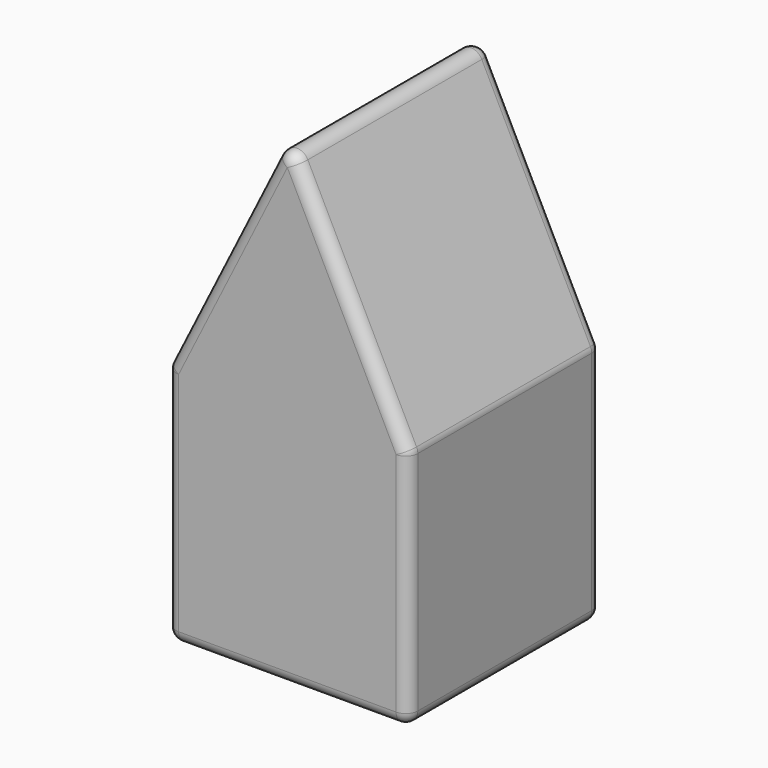
from build123d import *

# Parameters (mm, degrees)
F0_W     = 101.6
F0_H     = 101.6
F1_DEPTH = 101.6
F2_W     = 101.6
F2_H     = 101.6
F3_DEPTH = 101.6
F5_DEPTH = 101.6
F6_R     = 5.08


with BuildPart() as f1:
    # F0 (on Top) → F1 (new body)
    with BuildSketch(Plane.XY):
        Rectangle(F0_W, F0_H)
    extrude(amount=F1_DEPTH)

    # F2 (on face) → F3 (join)
    with BuildSketch(Plane.XY.offset(101.6)):
        Rectangle(F2_W, F2_H)
    extrude(amount=F3_DEPTH)

    # F4 (on face) → F5 (cut)
    with BuildSketch(Plane(origin=(0, 50.8, 0), x_dir=(-1, 0, 0), z_dir=(0, 1, 0))):
        Polygon((-50.8, 101.6), (0, 203.2), (-50.8, 203.2), align=None)
        Polygon((50.8, 203.2), (0, 203.2), (50.8, 101.6), align=None)
    extrude(amount=-F5_DEPTH, mode=Mode.SUBTRACT)

    # F6
    f6_edges = [f1.edges().sort_by_distance(p)[0] for p in [
        (25.4, 50.8, 152.4),
        (50.8, 0, 101.6),
        (50.8, 50.8, 50.8),
        (0, 0, 203.2),
        (-50.8, 0, 101.6),
        (-50.8, 50.8, 50.8),
        (-50.8, 0, 0),
        (0, 50.8, 0),
        (-50.8, -50.8, 50.8),
        (50.8, -50.8, 50.8),
        (-25.4, -50.8, 152.4),
        (-25.4, 50.8, 152.4),
        (0, -50.8, 0),
        (50.8, 0, 0),
        (25.4, -50.8, 152.4),
    ]]
    fillet(f6_edges, radius=F6_R)


solid = f1.part
